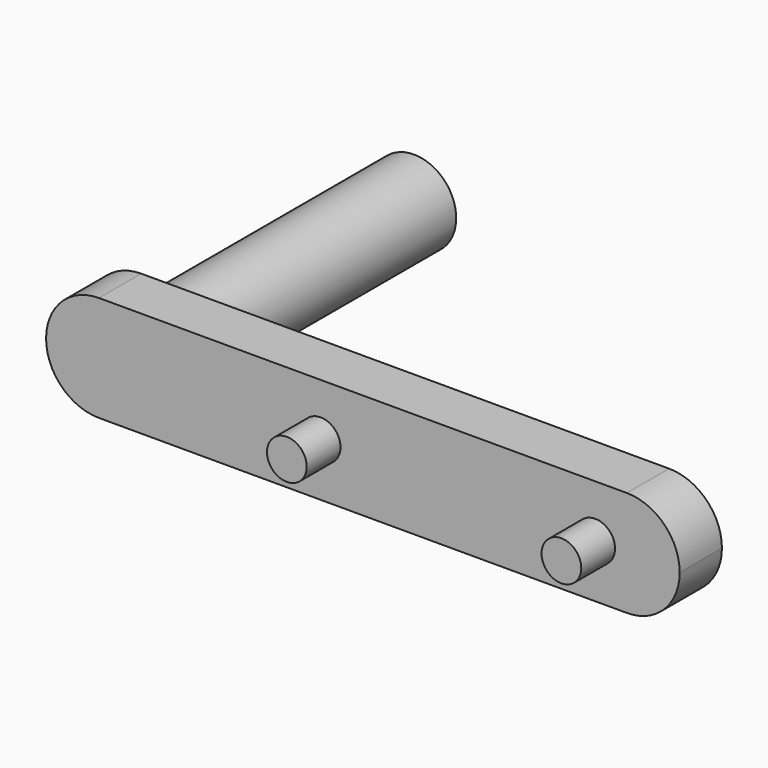
from build123d import *

# Parameters (mm, degrees)
F0_W     = 38.1
F0_H     = 6.35
F1_DEPTH = 3.175
F2_R     = 1.1938
F3_DEPTH = 2.54
F4_R     = 2.54
F5_DEPTH = 18.415
F6_R     = 3.17499


# Not quite as in the source:
# - a fillet or chamfer is up to 0.001 mm smaller than in the source, because OpenCascade refuses the exact size


with BuildPart() as f1:
    # F0 (on Front) → F1 (new body)
    with BuildSketch(Plane.XZ):
        with Locations((19.05, 3.175)):
            Rectangle(F0_W, F0_H)
    extrude(amount=F1_DEPTH)

    # F2 (on face) → F3 (join)
    with BuildSketch(Plane.XZ.offset(3.175)):
        with Locations((16.51, 3.175)):
            Circle(F2_R)
        with Locations((33.02, 3.175)):
            Circle(F2_R)
    extrude(amount=F3_DEPTH)

    # F4 (on face) → F5 (join)
    with BuildSketch(Plane(origin=(0, 0, 0), x_dir=(-1, 0, 0), z_dir=(0, 1, 0))):
        with Locations((-4.8514, 3.175)):
            Circle(F4_R)
    extrude(amount=F5_DEPTH)

    # F6 (radius 3.175 in the source; OpenCascade refuses exactly that, so slightly less here)
    f6_edges = [f1.edges().sort_by_distance(p)[0] for p in [
        (38.1, -1.5875, 6.35),
        (38.1, -1.5875, 0),
        (0, -1.5875, 6.35),
        (0, -1.5875, 0),
    ]]
    fillet(f6_edges, radius=F6_R)


solid = f1.part
